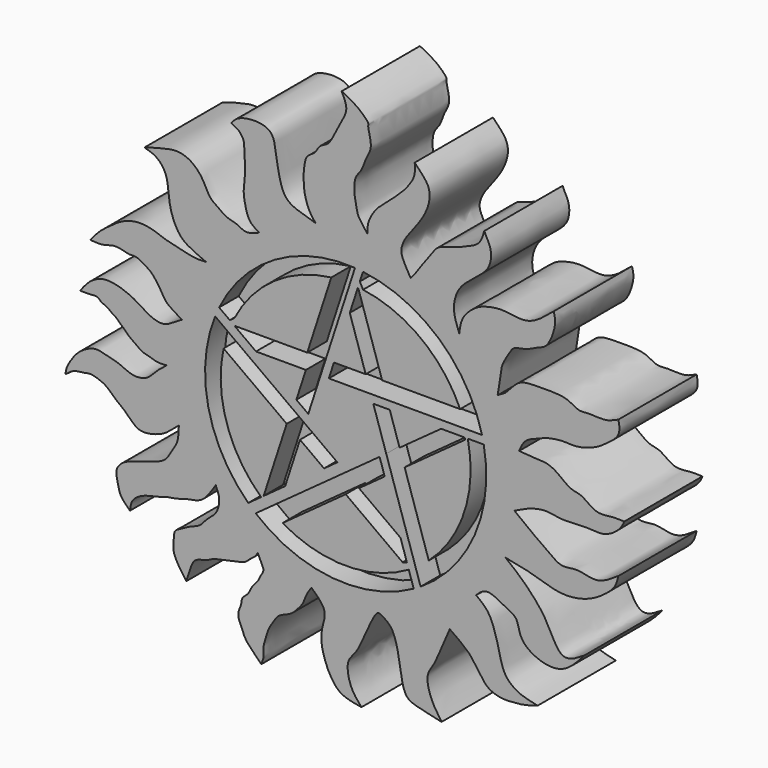
from build123d import *

# Parameters (mm, degrees)
F1_DEPTH = 6.35
F3_DEPTH = 1.5875


# Not quite as in the source:
# - a length typed as a fraction of an inch, garbled in the dataset ("3 / 203.2 mm" for 3/8 in), is restored


with BuildPart() as f1:
    # F0 (on Front) → F1 (new body)
    with BuildSketch(Plane.XZ):
        with BuildLine():
            add(Edge.make_bspline(
                [(18.8331263454, 36.3106213719), (18.9928966431, 35.9981643243), (19.3018797444, 35.3938971421), (18.8208643925, 34.5899386637), (18.547484939, 34.0224293639), (18.2576525022, 33.4811901482), (17.9596670729, 32.9400655765), (17.3618543962, 32.7817352013), (17.1697281027, 32.2242380648), (16.6675285403, 31.9705213642), (16.4670462701, 31.6771475738), (16.3573443652, 30.8523657582), (16.3751181829, 30.2996906452), (16.4126206359, 29.6820470846), (16.6833850627, 28.8045665841), (16.9978601115, 28.4128579434), (17.147121951, 28.2269380987)],
                knots=[0, 0, 0, 0, 0.0874382698, 0.1690986884, 0.2400607005, 0.3092556695, 0.3773002458, 0.4432865801, 0.5087271415, 0.5726214643, 0.6245098455, 0.7038948725, 0.7708309715, 0.8397909787, 0.9239586946, 1, 1, 1, 1], degree=3))
            add(Edge.make_bspline(
                [(17.147121951, 28.2269380987), (16.7356547423, 28.3413143893), (15.9712689538, 28.5537921015), (15.0987121487, 29.0013553838), (14.7577922109, 30.1957034719), (14.5791213212, 31.2982171402), (14.4213094926, 32.5260795141), (13.547552027, 32.80574844), (12.7851821815, 32.7966530481), (12.0047389931, 32.5862030682), (11.7741739493, 32.2908253548), (11.6702597588, 32.1577005088)],
                knots=[0, 0, 0, 0, 0.1282974811, 0.2383392145, 0.3623226769, 0.4886698804, 0.6108209922, 0.7131268021, 0.8154896024, 0.916842344, 1, 1, 1, 1], degree=3))
            add(Edge.make_bspline(
                [(11.6702597588, 32.1577005088), (11.7883666701, 32.1037788333), (12.0127064376, 32.0013565785), (12.2559568148, 31.8154282848), (12.5106570632, 31.4390040822), (12.5230684239, 30.9182924902), (12.5658481324, 30.1851211574), (12.5664601139, 29.2763415312), (12.4290930054, 28.4933686833), (12.5918578245, 27.6768216263), (12.8216658836, 26.8661456772), (13.2799046616, 26.6187290589), (13.5046150535, 26.4974012971)],
                knots=[0, 0, 0, 0, 0.0774611957, 0.1471347142, 0.2296238116, 0.3198991215, 0.4289318391, 0.5500077217, 0.662594825, 0.7779010749, 0.8910874878, 1, 1, 1, 1], degree=3))
            add(Edge.make_bspline(
                [(13.5046150535, 26.4974012971), (13.1859265689, 26.3656418151), (12.6052470252, 26.1255639975), (12.0647141709, 26.5544187455), (11.3228686086, 26.6491763091), (10.9016133155, 27.0408079115), (10.2575580062, 27.3937498359), (9.9675112819, 28.1514911538), (9.3894838197, 28.969940218), (8.4046146452, 29.5100383246), (7.1945583467, 29.2975280238), (6.4246158135, 29.0562194865), (6.0361661017, 28.9344750345)],
                knots=[0, 0, 0, 0, 0.1034133745, 0.1884286192, 0.2793764848, 0.3604811336, 0.4500780147, 0.5456137691, 0.6528255571, 0.7634531392, 0.8806578986, 1, 1, 1, 1], degree=3))
            add(Edge.make_bspline(
                [(6.0361661017, 28.9344750345), (6.3090211941, 28.8599191708), (6.8770075852, 28.7047206163), (7.5403104355, 27.85354386), (7.5797351418, 26.7225012846), (7.7905858311, 25.637973419), (8.2666399326, 24.6696835109), (8.9081762528, 24.1765286463), (9.6383431981, 23.8664064516), (10.045543313, 23.6934572458)],
                knots=[0, 0, 0, 0, 0.1305716366, 0.2718032931, 0.4216934421, 0.5722406722, 0.7163482936, 0.8418128783, 1, 1, 1, 1], degree=3))
            add(Edge.make_bspline(
                [(10.045543313, 23.6934572458), (9.8113775927, 23.6807901244), (9.3160108392, 23.6539934147), (8.4575514647, 23.8757927447), (7.5153442627, 24.0606263987), (6.8280263149, 24.3572498097), (6.0837483741, 24.5387359926), (5.3251189102, 24.5280562079), (4.4789374211, 24.2356630504), (3.7573142515, 23.6899578771), (3.1053039005, 23.2238857817), (2.725109332, 22.7532988362), (2.5285636075, 22.5100237876)],
                knots=[0, 0, 0, 0, 0.0929310561, 0.1965913521, 0.3043581007, 0.3994841275, 0.4944082504, 0.5894793284, 0.6926105158, 0.7968836409, 0.8949967852, 1, 1, 1, 1], degree=3))
            add(Edge.make_bspline(
                [(2.5285636075, 22.5100237876), (2.8184147257, 22.4851417659), (3.3938870749, 22.4357408334), (4.1650935086, 22.8065154349), (5.0574631758, 22.4399401684), (5.4620812724, 22.5745799723), (5.9724346303, 22.2709714539), (6.4551052339, 22.0026449595), (6.8010425381, 21.5701989117), (7.0698858531, 21.1922976943), (7.3831363474, 20.591752799), (7.7414165155, 20.3236955412), (8.0826132144, 20.1154758437), (8.3423104683, 19.9666046365), (8.4770750254, 19.8893509805)],
                knots=[0, 0, 0, 0, 0.1014358569, 0.2013914289, 0.3049756965, 0.3740277223, 0.4554246303, 0.5384369993, 0.6184255736, 0.6944352164, 0.7839174037, 0.8569613469, 0.9257730282, 1, 1, 1, 1], degree=3))
            add(Edge.make_bspline(
                [(8.4770750254, 19.8893509805), (8.26535853, 19.770882288), (7.8594962194, 19.5437768035), (7.346207607, 19.1641329073), (6.450106196, 19.3437044675), (5.657823891, 19.9196049686), (4.7636060334, 20.3671298382), (3.4844958376, 20.7029025993), (2.4578556936, 20.1931670391), (2.0599192501, 19.6578466958), (1.8652869925, 19.3960194402)],
                knots=[0, 0, 0, 0, 0.1098457495, 0.2105752298, 0.3296287584, 0.4585773297, 0.5898352555, 0.7364998651, 0.8711210623, 1, 1, 1, 1], degree=3))
            add(Edge.make_bspline(
                [(1.8652869925, 19.3960194402), (2.0082753726, 19.3974985826), (2.2683052796, 19.4001884604), (2.5142990305, 19.3811529563), (3.0215440914, 19.4648612809), (3.1733512663, 19.1799423809), (3.6285728374, 19.0539602168), (3.858869738, 18.8108901275), (4.2379380731, 18.6201442681), (4.3960943152, 18.3986423311), (4.7095754263, 18.1863185582), (4.9518318048, 17.8621114647), (5.3084258659, 17.636333021), (5.6323706948, 17.3952339687), (5.9240458325, 17.1724210278), (6.4404215063, 17.0886523717), (6.8319658867, 16.9133277385), (7.2519155125, 16.9398940845), (7.4834804982, 16.954543069)],
                knots=[0, 0, 0, 0, 0.0626853758, 0.1139957837, 0.1810559701, 0.2339302949, 0.2999632213, 0.358564209, 0.421773997, 0.4734954729, 0.5336146021, 0.5969705458, 0.661480987, 0.7243952871, 0.7843432225, 0.8548917384, 0.9199856591, 1, 1, 1, 1], degree=3))
            add(Edge.make_bspline(
                [(7.4834804982, 16.954543069), (7.2612196875, 16.7854233828), (6.8129298021, 16.4443167139), (6.2560954433, 15.7345084489), (5.2669766127, 15.5894659528), (4.4583774952, 16.0636324377), (3.5513136305, 16.2659039879), (2.7589634854, 16.4986166887), (1.8207299294, 15.9457893755), (1.4332967241, 15.4899498856), (0.9608301409, 14.7790120313), (0.9278264472, 14.4534709831), (0.9137363522, 14.3144894391)],
                knots=[0, 0, 0, 0, 0.102074293, 0.2058791785, 0.3112937303, 0.4181902206, 0.5250867776, 0.6245281404, 0.7355878114, 0.8245841687, 0.9251106329, 1, 1, 1, 1], degree=3))
            add(Edge.make_bspline(
                [(0.9137363522, 14.3144894391), (1.1008989531, 14.4654994114), (1.4609195796, 14.7559778754), (2.0887444184, 14.7507845593), (2.5217694198, 14.914680953), (3.1724207297, 14.6917156718), (3.6178577639, 14.4860456437), (4.1024812457, 13.958144068), (4.6844200002, 13.5665162469), (5.1527359956, 13.0781667027), (5.6096454858, 12.654796117), (6.3236143084, 12.6349190159), (7.2798326747, 12.9289850931), (7.8133155428, 13.3982735677), (8.1214649436, 13.6554438824), (8.2677509636, 13.7775288895)],
                knots=[0, 0, 0, 0, 0.079458853, 0.1528447772, 0.2170878682, 0.2938886049, 0.3615038526, 0.4409881257, 0.5216806244, 0.6002218221, 0.6731824479, 0.7517739975, 0.8468814349, 0.9273108907, 1, 1, 1, 1], degree=3))
            add(Edge.make_bspline(
                [(8.2677509636, 13.7775288895), (8.2730364941, 13.4050117419), (8.217602118, 12.7222569327), (7.8238786666, 12.2552906743), (7.4787350096, 11.4689696153), (6.6509739527, 11.1884311656), (6.0014336392, 10.9660207565), (5.270011968, 10.7500085351), (4.6373159397, 10.5313233479), (4.1068180636, 9.953526866), (4.3259976144, 9.1777260242), (4.434243058, 8.5023223643), (4.8690224655, 8.0940894399), (5.1008788869, 7.8763896599)],
                knots=[0, 0, 0, 0, 0.106202297, 0.1869060438, 0.28038459, 0.3754216672, 0.4629656104, 0.5533904317, 0.639151387, 0.7256780269, 0.8157823539, 0.9013703539, 1, 1, 1, 1], degree=3))
            add(Edge.make_bspline(
                [(5.1008788869, 7.8763896599), (5.1310516166, 8.1000161086), (5.160259873, 8.5919064758), (6.0368632119, 9.1051217214), (6.8359959065, 9.2012253064), (7.4661432042, 9.4687532543), (8.1874229164, 9.5269975353), (8.745644715, 9.7691525371), (9.6985638664, 9.8529633397), (10.2346809952, 10.491879994), (10.5226594671, 10.9253915483), (10.6660984457, 11.1413178965)],
                knots=[0, 0, 0, 0, 0.1038910509, 0.2264035756, 0.3416702482, 0.4463923887, 0.5525628185, 0.6526696211, 0.7737497835, 0.8874116541, 1, 1, 1, 1], degree=3))
            add(Edge.make_bspline(
                [(10.6660984457, 11.1413178965), (10.7527569416, 10.9524171747), (10.9302473223, 10.5655012293), (10.8589886453, 9.841427682), (10.5531984588, 9.3661608715), (10.0090327309, 8.9834051884), (9.6976655246, 8.4614432571), (8.9220973428, 8.2404286334), (8.5114137935, 7.9479087987), (7.9235196015, 7.7293015269), (7.9714533074, 7.1573647868), (7.8704640984, 6.7143780756), (8.0058494653, 6.1293606719), (8.4715216146, 5.4265043037), (8.6676470809, 5.1505600257), (8.7518971413, 5.032022018)],
                knots=[0, 0, 0, 0, 0.0789722026, 0.1617560171, 0.2359239628, 0.3158952106, 0.3926986646, 0.4795035795, 0.5524742294, 0.625666678, 0.6959465546, 0.7630582728, 0.8393476535, 0.9309883059, 1, 1, 1, 1], degree=3))
            add(Edge.make_bspline(
                [(8.7518971413, 5.032022018), (8.804964072, 5.2060582538), (8.9082393486, 5.5447573306), (9.052994233, 5.9927378592), (9.3161765445, 6.5417239279), (10.0778761313, 6.6144700115), (10.4922820233, 6.9174908032), (11.1548486707, 7.0053302642), (11.5743454541, 7.1137834486), (12.0829396787, 7.2321979702), (12.6152395035, 7.3395409019), (12.8501356621, 7.6626061271), (13.2357323086, 7.8702494318), (13.337345244, 8.0764537195), (13.3849624544, 8.1730838865)],
                knots=[0, 0, 0, 0, 0.0862271269, 0.1678101426, 0.2553192883, 0.3540112288, 0.4394005821, 0.5337394389, 0.6122658197, 0.6976654615, 0.7829423656, 0.8560732516, 0.932553966, 1, 1, 1, 1], degree=3))
            add(Edge.make_bspline(
                [(13.3849624544, 8.1730838865), (13.4608598972, 7.9967257476), (13.6005792035, 7.6720687376), (13.8445025485, 7.2889281832), (13.5525097885, 6.9153929809), (13.4197820619, 6.5188631253), (12.9836877132, 6.1393847341), (12.8014231608, 5.5665962948), (12.3275621379, 5.3084250089), (12.3545621075, 4.834685755), (12.0277705269, 4.3025507517), (12.2837797153, 3.6550571418), (12.5651054497, 2.9871621328), (12.9150445674, 2.585764995), (13.3611965934, 2.1339604596), (13.6205423623, 1.8713289173)],
                knots=[0, 0, 0, 0, 0.0774710257, 0.142616109, 0.2089966971, 0.2760794555, 0.3532654092, 0.4325825219, 0.5035676882, 0.5708315564, 0.6493442383, 0.7337054785, 0.8210574628, 0.8959816672, 1, 1, 1, 1], degree=3))
            add(Edge.make_bspline(
                [(13.6205423623, 1.8713289173), (13.690510337, 2.0441436044), (13.8314818751, 2.3923307906), (13.7228455127, 2.9760384181), (13.936715855, 3.4652967039), (14.031002713, 3.9842540525), (14.459560892, 4.662661032), (14.7489996698, 5.0661737234), (15.2561520569, 5.2381994842), (15.6601190115, 5.4412780225), (15.9556287761, 5.7833525458), (16.3264320717, 6.1686586037), (16.4891680483, 6.6806623169), (16.6927505474, 7.0525812614), (16.8204290924, 7.2281902987), (16.8793946505, 7.3092915118)],
                knots=[0, 0, 0, 0, 0.0803661611, 0.1619218133, 0.2390867546, 0.3180751187, 0.4142293525, 0.4902024999, 0.567343173, 0.6396974695, 0.7117373362, 0.7904574494, 0.8696053903, 0.9397800866, 1, 1, 1, 1], degree=3))
            add(Edge.make_bspline(
                [(16.8793946505, 7.3092915118), (17.2703157102, 6.9481049704), (18.0629485115, 6.2157619743), (17.1658125399, 4.742159561), (18.2311341194, 2.0569507369), (19.2900466517, 1.6724225497), (19.8567322641, 1.5763897233), (20.1220978051, 1.5314198099)],
                knots=[0, 0, 0, 0, 0.1989041253, 0.4032986458, 0.6768369906, 0.8486703651, 1, 1, 1, 1], degree=3))
            add(Edge.make_bspline(
                [(20.1220978051, 1.5314198099), (19.862211626, 1.8296524056), (19.3305336402, 2.4397799096), (19.0963313757, 4.0247639409), (19.9780497263, 4.4990689679), (20.9639462951, 7.4392506636), (21.3155546001, 7.2683737319), (21.3982388377, 7.2281902987)],
                knots=[0, 0, 0, 0, 0.202180779, 0.4136236475, 0.5993251298, 0.905777265, 1, 1, 1, 1], degree=3))
            add(Edge.make_bspline(
                [(21.3982388377, 7.2281902987), (21.6500728753, 7.0798246662), (22.2732756251, 6.7126425109), (22.6317260576, 4.7493347526), (22.8729720768, 3.014429211), (23.7704315003, 2.7285637023), (24.7442728889, 2.5103317633), (25.3236134029, 2.3821811192)],
                knots=[0, 0, 0, 0, 0.1641885448, 0.4067555081, 0.6278763242, 0.7803602953, 1, 1, 1, 1], degree=3))
            add(Edge.make_bspline(
                [(25.3236134029, 2.3821811192), (25.0954354119, 2.7103232383), (24.6333238251, 3.3748845954), (24.2519402276, 4.7634931067), (24.8494160691, 5.4461232155), (25.3230379772, 6.6622471122), (25.6768111468, 7.4575926784), (25.8553389884, 7.8589553013)],
                knots=[0, 0, 0, 0, 0.2041113903, 0.4133713248, 0.5805800915, 0.7883442345, 1, 1, 1, 1], degree=3))
            add(Edge.make_bspline(
                [(25.8553389884, 7.8589553013), (26.0105812403, 7.7571894201), (26.3596929279, 7.5283363977), (27.1212936034, 6.9078323221), (27.3896392154, 6.5364570775), (27.7979839755, 5.9418197215), (28.0759844908, 5.5641850265), (28.4015539382, 5.2430510023), (29.0919491859, 4.9802732005), (29.8872994967, 4.9885036612), (30.7560736815, 5.0842989575), (31.2916903993, 5.2537626063), (31.5569974482, 5.3377030417)],
                knots=[0, 0, 0, 0, 0.0950865333, 0.2138323795, 0.2985947797, 0.4001142276, 0.4838062009, 0.5640389505, 0.6664041781, 0.775385945, 0.8887419117, 1, 1, 1, 1], degree=3))
            add(Edge.make_bspline(
                [(27.5662578642, 10.3580662981), (27.8407987121, 10.149711996), (28.4047756654, 9.7216990961), (28.8118664277, 8.6234617101), (29.0812895551, 7.5998030231), (29.263238336, 6.7206351143), (29.6864116848, 6.0605248419), (30.3671660759, 5.6406994498), (30.8688592019, 5.4994817367), (31.3165069548, 5.3942414457), (31.5569974482, 5.3377030417)],
                knots=[0, 0, 0, 0, 0.1374622425, 0.2823825208, 0.4231579826, 0.5505764157, 0.6693222279, 0.78806794, 0.8861434122, 1, 1, 1, 1], degree=3))
            add(Edge.make_bspline(
                [(27.5662578642, 10.3580662981), (27.7770141163, 10.5625079593), (28.243845541, 11.0151934381), (29.3683068006, 10.3161288175), (30.3614197142, 9.9489793409), (30.2966266943, 8.4709841104), (32.9921564745, 7.341053168), (34.0561718744, 8.5758665333), (34.5850363374, 9.1882701963)],
                knots=[0, 0, 0, 0, 0.1270349227, 0.2811720323, 0.419227983, 0.5737209603, 0.788772509, 1, 1, 1, 1], degree=3))
            add(Edge.make_bspline(
                [(34.5850363374, 9.1882701963), (34.1057889944, 8.8854947079), (33.148340547, 8.2805571851), (32.3796898738, 9.9114878695), (31.8260046548, 10.8999212004), (30.6286241278, 12.2127873322), (29.8482409137, 12.8274493253), (29.4710722245, 13.1230400875)],
                knots=[0, 0, 0, 0, 0.1974671089, 0.3943019678, 0.5793110377, 0.7972455615, 1, 1, 1, 1], degree=3))
            add(Edge.make_bspline(
                [(29.4710722245, 13.1230400875), (29.9658261188, 13.0330340645), (30.9087475757, 12.8614970411), (32.0508887052, 12.4668576847), (33.3273971843, 12.1572896497), (34.79263733, 12.3948264313), (35.8946239496, 13.0782187758), (36.633751448, 13.7321826454), (36.7477645072, 14.2242369161), (36.800621141, 14.4523540512)],
                knots=[0, 0, 0, 0, 0.1592644531, 0.3035324671, 0.4530088647, 0.6117286891, 0.7619045428, 0.889618571, 1, 1, 1, 1], degree=3))
            add(Edge.make_bspline(
                [(36.800621141, 14.4523540512), (36.3202969228, 14.1277601799), (35.4173898731, 13.5175929563), (34.158502147, 14.0703587685), (33.090876465, 13.6780014423), (32.1098291727, 14.4893965006), (30.9979629158, 15.2314924878), (30.3578600287, 15.7453668397), (30.0477054606, 15.9943588078)],
                knots=[0, 0, 0, 0, 0.1875159533, 0.3524899844, 0.5019059303, 0.6624080752, 0.8364236754, 1, 1, 1, 1], degree=3))
            add(Edge.make_bspline(
                [(30.0477054606, 15.9943588078), (30.3531835419, 16.1475825041), (30.9792132331, 16.4619065212), (32.1430408045, 16.7287795994), (33.125157231, 16.4138601089), (34.6543291432, 16.6306215778), (35.8657198374, 16.3873105913), (36.8407789581, 17.0481609028), (37.1089891836, 17.4834733869), (37.180095911, 17.68944785)],
                knots=[0, 0, 0, 0, 0.1400300415, 0.2857862834, 0.4237535201, 0.5921473053, 0.7434110314, 0.8854231971, 1, 1, 1, 1], degree=3))
            add(Edge.make_bspline(
                [(37.180095911, 17.68944785), (36.9195653743, 17.7016983601), (36.3787534773, 17.7298210614), (35.3187000407, 17.5031589118), (34.474267773, 18.3584419577), (33.6822808997, 18.3330899023), (32.8315784113, 19.1275689409), (32.1248517767, 19.4136342155), (31.5975440096, 19.4104846608), (30.7965724668, 19.466242823), (30.3578600287, 19.5041820407)],
                knots=[0, 0, 0, 0, 0.1184868028, 0.2516808047, 0.3890699928, 0.5034964262, 0.6437633197, 0.7569569738, 0.8518105356, 1, 1, 1, 1], degree=3))
            add(Edge.make_bspline(
                [(30.3578600287, 19.5041820407), (30.4718473248, 19.7695982602), (30.6978926176, 20.3077600771), (31.5908393059, 20.5934782), (32.1026939766, 20.8406630881), (33.1689982982, 21.0437730661), (34.1254177527, 20.8825672814), (35.4091381417, 21.3232440109), (36.0492318408, 21.8038279252), (36.9733586187, 22.4738736556), (36.8624655959, 23.1049589693), (36.800621141, 23.3909990638)],
                knots=[0, 0, 0, 0, 0.1064362396, 0.2140112336, 0.3034008649, 0.4208671062, 0.5374976353, 0.6688668376, 0.7761807692, 0.8931066139, 1, 1, 1, 1], degree=3))
            add(Edge.make_bspline(
                [(36.800621141, 23.3909990638), (36.5338211532, 23.2747811216), (36.031486993, 23.0042358719), (34.8712064009, 23.1556045913), (34.2254003613, 23.0142455896), (33.6203458498, 23.449130949), (32.860997458, 23.6058573419), (31.4758275322, 23.5768787185), (30.2759939853, 23.5685941909), (29.7765404009, 22.8240268764), (29.4710722245, 22.5428044796)],
                knots=[0, 0, 0, 0, 0.1179215868, 0.253451167, 0.3554742476, 0.4596253219, 0.5718826527, 0.7226574632, 0.8586384439, 1, 1, 1, 1], degree=3))
            add(Edge.make_bspline(
                [(29.4710722245, 22.5428044796), (29.2867479649, 22.4148016423), (29.1494193176, 22.3619956523), (28.9650950581, 22.233992815)],
                knots=[0, 0, 0, 0, 0.5927710663, 0.5927710663, 0.5927710663, 0.5927710663], degree=3))
            add(Edge.make_bspline(
                [(28.9650950581, 22.233992815), (29.0156186663, 22.6354114876), (29.1752157866, 23.3888716604), (29.2012874667, 24.1101486497), (29.7626601416, 24.9331235233), (29.9944059062, 25.3587964515), (30.8379958274, 25.4002277235), (31.5486035988, 25.851772768), (32.2291612465, 25.9662535362), (32.8145692511, 27.5102738675), (32.6528182744, 28.0085552384), (32.6027710415, 28.2121840864)],
                knots=[0, 0, 0, 0, 0.1312255294, 0.2352236923, 0.3534108751, 0.434524181, 0.5410529487, 0.6518037498, 0.7485993587, 0.8971736949, 1, 1, 1, 1], degree=3))
            add(Edge.make_bspline(
                [(32.6027710415, 28.2121840864), (32.2650676488, 27.9235539976), (31.6248119985, 27.3763369745), (30.6297378955, 26.9570490609), (29.2966985595, 27.2825079743), (28.3508942064, 27.0932802371), (27.6121966473, 26.889194726), (26.5941413493, 26.0107047074), (26.5129841864, 25.2870608062), (26.4741842128, 24.941097945)],
                knots=[0, 0, 0, 0, 0.1556201025, 0.2950418979, 0.4533220538, 0.5863259312, 0.7060593453, 0.8594715581, 1, 1, 1, 1], degree=3))
            add(Edge.make_bspline(
                [(26.4741842128, 24.941097945), (26.3514002431, 25.2665963264), (26.1232116319, 25.8715207626), (26.1079447677, 26.6247033143), (26.3952204071, 27.5666751203), (27.2990877502, 28.3519298989), (28.0617891584, 28.9031030136), (28.5345071537, 29.5223314194), (28.5684520315, 30.4498832764), (28.2497271227, 31.0071049361), (28.1450204495, 31.2415160484), (28.1002279371, 31.3417948782)],
                knots=[0, 0, 0, 0, 0.12341415, 0.2293597738, 0.3493894416, 0.4844956503, 0.604971743, 0.7117938749, 0.828132733, 0.9264768285, 1, 1, 1, 1], degree=3))
            add(Edge.make_bspline(
                [(28.1002279371, 31.3417948782), (28.0155610557, 31.0632302729), (27.8555598889, 30.5368064675), (27.2535561442, 30.1977105228), (26.4769781998, 29.8839410302), (25.6537634522, 29.6408072902), (24.9644761985, 29.4245707239), (24.5588626913, 28.6975264884), (24.0032548159, 28.0397630048), (23.690483014, 27.534849587), (23.4422131978, 27.2336626261), (23.3190301806, 27.0842239261)],
                knots=[0, 0, 0, 0, 0.1166396345, 0.220422405, 0.3391775888, 0.4597426261, 0.56626386, 0.6820133865, 0.802530431, 0.9020223332, 1, 1, 1, 1], degree=3))
            add(Edge.make_bspline(
                [(23.3190301806, 27.0842239261), (23.207392713, 27.2785419521), (22.9799732415, 27.6743920528), (22.6298717134, 28.3686287165), (22.8249366164, 29.014669868), (23.1830708087, 29.5763216647), (23.6314986007, 30.1258282768), (24.2003994607, 30.9142747662), (24.5837622944, 31.8490541075), (24.5591142752, 32.7962645029), (23.8110774741, 33.5203458836), (23.6431550864, 33.7097539968), (23.5815271735, 33.7792672217)],
                knots=[0, 0, 0, 0, 0.0960358446, 0.195637016, 0.2876124497, 0.3812781974, 0.478641203, 0.5926855625, 0.7085007648, 0.8185096777, 0.9333926231, 1, 1, 1, 1], degree=3))
            add(Edge.make_bspline(
                [(23.5815271735, 33.7792672217), (23.5965171071, 33.5308544569), (23.6250154996, 33.0585798825), (23.3173381804, 32.5190278505), (22.9052832524, 31.9476567004), (21.9182945274, 31.048432167), (21.1894725228, 30.4654958604), (20.7746274811, 29.8800019699), (20.4957998604, 29.2717636541), (20.5159606597, 28.8750241994), (20.5257572276, 28.6822399281)],
                knots=[0, 0, 0, 0, 0.1209034567, 0.2298578682, 0.3504254691, 0.5161820755, 0.6562102151, 0.7758169804, 0.891064628, 1, 1, 1, 1], degree=3))
            add(Edge.make_bspline(
                [(20.5257572276, 28.6822399281), (20.3372928323, 28.9702435974), (19.9127607057, 29.4232376119), (19.7972213064, 29.9732492001), (19.6865645412, 30.5036921469), (19.6303232412, 31.1506152458), (19.7454082425, 31.8204144231), (20.1778443205, 32.1940991035), (20.3710357113, 33.0121296425), (20.9153128604, 33.714631346), (20.4885118921, 34.861740537), (20.6524727837, 35.0574623831), (19.9458763548, 35.7060867041), (19.566352196, 35.9116388276), (19.1392282605, 36.1950769301), (18.8331263454, 36.3106213719)],
                knots=[0, 0, 0, 0, 0.0924262416, 0.1613196835, 0.229847587, 0.3062078219, 0.3816823434, 0.450737597, 0.5348653024, 0.6234608306, 0.7212096806, 0.762302857, 0.8486178567, 0.9145392041, 1, 1, 1, 1], degree=3))
        make_face()
    extrude(amount=-F1_DEPTH)

    # F2 (on face) → F3 (cut)
    with BuildSketch(Plane.XZ):
        with BuildLine():
            Line((15.8990849661, 17.7291133536), (16.6707787888, 17.1684449728))
            Line((16.6707787888, 17.1684449728), (17.4715995585, 19.633117872))
            Line((17.4715995585, 19.633117872), (19.7028291929, 26.5001365854))
            ThreePointArc((19.7028291929, 26.5001365854), (14.5106993886, 25.2828586964), (10.8850449131, 21.3720266892))
            Line((10.8850449131, 21.3720266892), (11.5767224806, 20.8694935207))
            Line((11.5767224806, 20.8694935207), (11.874861371, 21.0807859455))
            ThreePointArc((11.874861371, 21.0807859455), (14.4709899326, 24.0540728832), (18.1631350921, 25.4499177325))
            Line((18.1631350921, 25.4499177325), (16.6032606598, 20.649117872))
            Line((16.6032606598, 20.649117872), (11.8800435393, 20.649117872))
            Line((11.8800435393, 20.649117872), (13.2784475705, 19.633117872))
            Line((13.2784475705, 19.633117872), (16.5177335358, 19.633117872))
            Line((16.5177335358, 19.633117872), (15.8990849661, 17.7291133536))
        make_face()
        with BuildLine():
            Line((17.6948176556, 14.3882781441), (18.5590788769, 15.0162006766))
            Line((18.5590788769, 15.0162006766), (16.4656611214, 16.5371577049))
            Line((16.4656611214, 16.5371577049), (10.6242261019, 20.7812086712))
            ThreePointArc((10.6242261019, 20.7812086712), (10.1770721106, 15.4688836478), (12.7737836756, 10.8129376758))
            Line((12.7737836756, 10.8129376758), (13.6104362638, 11.4208013623))
            ThreePointArc((13.6104362638, 11.4208013623), (11.3651745038, 14.9481366075), (11.1751170939, 19.125117872))
            Line((11.1751170939, 19.125117872), (15.2712814888, 16.1490802375))
            Line((15.2712814888, 16.1490802375), (13.7734537647, 11.5392405095))
            Line((13.7734537647, 11.5392405095), (15.1718577959, 12.5552405095))
            Line((15.1718577959, 12.5552405095), (16.1355427101, 15.5211577049))
            Line((16.1355427101, 15.5211577049), (17.6948176556, 14.3882781441))
        make_face()
        with BuildLine():
            Line((21.6308109598, 15.2071964386), (21.3006925484, 16.2231964386))
            Line((21.3006925484, 16.2231964386), (19.0992421402, 14.6237490938))
            Line((19.0992421402, 14.6237490938), (13.2578071207, 10.3796981275))
            ThreePointArc((13.2578071207, 10.3796981275), (18.2362280445, 8.3064960956), (23.5159317116, 9.4053913352))
            Line((23.5159317116, 9.4053913352), (23.1954065351, 10.3918663941))
            ThreePointArc((23.1954065351, 10.3918663941), (19.0992421402, 9.2816039869), (15.0030777454, 10.3918663941))
            Line((15.0030777454, 10.3918663941), (19.0992421402, 13.3679040287))
            Line((19.0992421402, 13.3679040287), (22.7967881874, 10.6814795761))
            Line((22.7967881874, 10.6814795761), (23.0722266914, 10.7709749711))
            Line((23.0722266914, 10.7709749711), (22.6612637252, 12.0357889267))
            Line((22.6612637252, 12.0357889267), (19.9635033615, 13.9958265612))
            Line((19.9635033615, 13.9958265612), (21.6308109598, 15.2071964386))
        make_face()
        with BuildLine():
            Line((21.9602295475, 19.125117872), (20.8919439277, 19.125117872))
            Line((20.8919439277, 19.125117872), (21.732823159, 16.5371577049))
            Line((21.732823159, 16.5371577049), (23.9640527934, 9.6701389915))
            ThreePointArc((23.9640527934, 9.6701389915), (27.474201766, 13.7642439913), (28.0606084461, 19.125117872))
            Line((28.0606084461, 19.125117872), (27.0520560443, 19.125117872))
            Line((27.0520560443, 19.125117872), (27.0342494198, 19.0745658462))
            ThreePointArc((27.0342494198, 19.0745658462), (26.8054762398, 14.8617672194), (24.491798367, 11.333750193))
            Line((24.491798367, 11.333750193), (22.9272027917, 16.1490802375))
            Line((22.9272027917, 16.1490802375), (26.8610563408, 19.0071921398))
            Line((26.8610563408, 19.0071921398), (26.8237106502, 19.125117872))
            Line((26.8237106502, 19.125117872), (25.2948447439, 19.125117872))
            Line((25.2948447439, 19.125117872), (22.5970843803, 17.1650802375))
            Line((22.5970843803, 17.1650802375), (21.9602295475, 19.125117872))
        make_face()
        with BuildLine():
            Line((18.3358607798, 20.649117872), (18.0057423684, 19.633117872))
            Line((18.0057423684, 19.633117872), (20.726884722, 19.633117872))
            Line((20.726884722, 19.633117872), (27.9472954923, 19.633117872))
            ThreePointArc((27.9472954923, 19.633117872), (25.1382659391, 24.2366159473), (20.2209815316, 26.4509229754))
            Line((20.2209815316, 26.4509229754), (20.0165222827, 25.8216621113))
            Line((20.0165222827, 25.8216621113), (20.2288580884, 25.4250728656))
            ThreePointArc((20.2288580884, 25.4250728656), (23.9997205145, 23.8564338765), (26.5281895695, 20.649117872))
            Line((26.5281895695, 20.649117872), (21.4650519304, 20.649117872))
            Line((21.4650519304, 20.649117872), (19.920472564, 25.4028443599))
            Line((19.920472564, 25.4028443599), (19.8804401462, 25.4028443599))
            Line((19.8804401462, 25.4028443599), (19.3663135452, 23.820525384))
            Line((19.3663135452, 23.820525384), (20.3967663106, 20.649117872))
            Line((20.3967663106, 20.649117872), (18.3358607798, 20.649117872))
        make_face()
    extrude(amount=-F3_DEPTH, mode=Mode.SUBTRACT)


solid = f1.part
